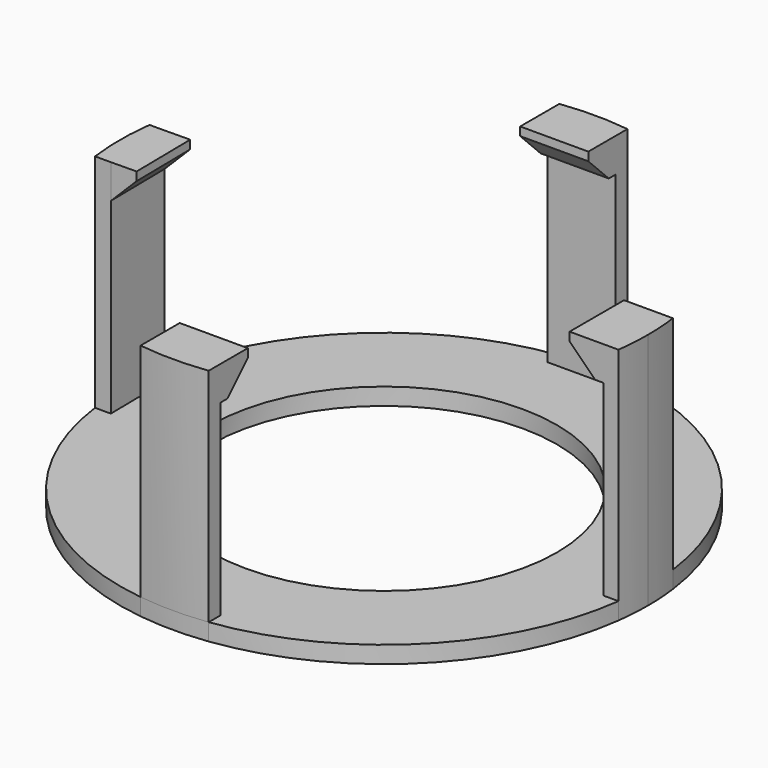
from build123d import *

# Parameters (mm, degrees)
F1_DEPTH  = 14
F0_R      = 10.15
F2_DEPTH  = 1
F3_W      = 4
F3_H      = 2
F4_DEPTH  = 2
F5_SIZE   = 1.5
F6_W      = 4
F6_H      = 2
F7_DEPTH  = 2
F8_SIZE   = 1.5
F9_W      = 4.0003886693
F9_H      = 2
F10_DEPTH = 1.5
F11_SIZE  = 1.49999
F12_W     = 4
F12_H     = 2
F13_DEPTH = 2
F14_SIZE  = 1.5


# Not quite as in the source:
# - a fillet or chamfer is up to 0.001 mm smaller than in the source, because OpenCascade refuses the exact size
# - a feature names something its author has since deleted; it is built from what else it names


with BuildPart() as f1:
    # F0 (on Top) → F1 (new body)
    with BuildSketch(Plane.XY):
        with BuildLine():
            Line((-14.4982938511, 2), (-15.3704261489, 2))
            ThreePointArc((-15.3704261489, 2), (-15.5, 0), (-15.3704261489, -2))
            Line((-15.3704261489, -2), (-14.4425309095, -2))
            Line((-14.4425309095, -2), (-14.4982938511, 2))
        make_face()
    extrude(amount=F1_DEPTH)

    # F9 (on face) → F10 (join)
    with BuildSketch(Plane(origin=(-14.4676006874, -0.2016889929, 0), x_dir=(-0.0139393809, 0.9999028421, 0), z_dir=(0.9999028421, 0.0139393809, 0))):
        with Locations((0.2017085905, 13)):
            Rectangle(F9_W, F9_H)
    extrude(amount=F10_DEPTH)

    # F11 (size 1.5 in the source; OpenCascade refuses exactly that, so slightly less here)
    f11_edges = [f1.edges().sort_by_distance(p)[0] for p in [
        (-12.970558, 0.020909, 12),
    ]]
    chamfer(f11_edges, length=F11_SIZE)


with BuildPart() as f1b:
    # F0 (on Top) → F1, piece 2 (new body)
    with BuildSketch(Plane.XY):
        with BuildLine():
            ThreePointArc((-2, -15.3704261489), (0, -15.5), (2, -15.3704261489))
            Line((2, -15.3704261489), (2, -14.4982938511))
            Line((2, -14.4982938511), (-2, -14.4982938511))
            Line((-2, -14.4982938511), (-2, -15.3704261489))
        make_face()
    extrude(amount=F1_DEPTH)

    # F3 (on face) → F4 (join)
    with BuildSketch(Plane(origin=(0, -14.4982938511, 0), x_dir=(-1, 0, 0), z_dir=(0, 1, 0))):
        with Locations((0, 13)):
            Rectangle(F3_W, F3_H)
    extrude(amount=F4_DEPTH)

    # F5
    f5_edges = [f1b.edges().sort_by_distance(p)[0] for p in [
        (0, -12.498294, 12),
    ]]
    chamfer(f5_edges, length=F5_SIZE)


with BuildPart() as f1c:
    # F0 (on Top) → F1, piece 3 (new body)
    with BuildSketch(Plane.XY):
        with BuildLine():
            Line((2, 14.4982938511), (2, 15.3704261489))
            ThreePointArc((2, 15.3704261489), (0, 15.5), (-2, 15.3704261489))
            Line((-2, 15.3704261489), (-2, 14.4982938511))
            Line((-2, 14.4982938511), (2, 14.4982938511))
        make_face()
    extrude(amount=F1_DEPTH)

    # F6 (on face) → F7 (join)
    with BuildSketch(Plane.XZ.offset(-14.4982938511)):
        with Locations((0, 13)):
            Rectangle(F6_W, F6_H)
    extrude(amount=F7_DEPTH)

    # F8
    f8_edges = [f1c.edges().sort_by_distance(p)[0] for p in [
        (0, 12.498294, 12),
    ]]
    chamfer(f8_edges, length=F8_SIZE)


with BuildPart() as f1d:
    # F0 (on Top) → F1, piece 4 (new body)
    with BuildSketch(Plane.XY):
        with BuildLine():
            ThreePointArc((15.3704261489, -2), (15.4675726167, -1.0020964753), (15.5, 0))
            ThreePointArc((15.5, 0), (15.4675726167, 1.0020964753), (15.3704261489, 2))
            Line((15.3704261489, 2), (14.4982938511, 2))
            Line((14.4982938511, 2), (14.4982938511, -2))
            Line((14.4982938511, -2), (15.3704261489, -2))
        make_face()
    extrude(amount=F1_DEPTH)

    # F12 (on face) → F13 (join)
    with BuildSketch(Plane(origin=(14.4982938511, 0, 0), x_dir=(0, -1, 0), z_dir=(-1, 0, 0))):
        with Locations((0, 13)):
            Rectangle(F12_W, F12_H)
    extrude(amount=F13_DEPTH)

    # F14
    f14_edges = [f1d.edges().sort_by_distance(p)[0] for p in [
        (12.498294, 0, 12),
    ]]
    chamfer(f14_edges, length=F14_SIZE)


with BuildPart() as f2:
    # F0 (on Top) → F2 (new body)
    with BuildSketch(Plane.XY):
        with BuildLine():
            Line((2, 14.4982938511), (2, 15.3704261489))
            ThreePointArc((2, 15.3704261489), (0, 15.5), (-2, 15.3704261489))
            Line((-2, 15.3704261489), (-2, 14.4982938511))
            Line((-2, 14.4982938511), (2, 14.4982938511))
        make_face()
        with BuildLine():
            Line((-14.4982938511, 2), (-15.3704261489, 2))
            ThreePointArc((-15.3704261489, 2), (-15.5, 0), (-15.3704261489, -2))
            Line((-15.3704261489, -2), (-14.4425309095, -2))
            Line((-14.4425309095, -2), (-14.4982938511, 2))
        make_face()
        with BuildLine():
            Line((14.4982938511, 2), (15.3704261489, 2))
            ThreePointArc((15.3704261489, 2), (10.9601551084, 10.9601551084), (2, 15.3704261489))
            Line((2, 15.3704261489), (2, 14.4982938511))
            Line((2, 14.4982938511), (-2, 14.4982938511))
            Line((-2, 14.4982938511), (-2, 15.3704261489))
            ThreePointArc((-2, 15.3704261489), (-10.9601551084, 10.9601551084), (-15.3704261489, 2))
            Line((-15.3704261489, 2), (-14.4982938511, 2))
            Line((-14.4982938511, 2), (-14.4425309095, -2))
            Line((-14.4425309095, -2), (-15.3704261489, -2))
            ThreePointArc((-15.3704261489, -2), (-10.9601551084, -10.9601551084), (-2, -15.3704261489))
            Line((-2, -15.3704261489), (-2, -14.4982938511))
            Line((-2, -14.4982938511), (2, -14.4982938511))
            Line((2, -14.4982938511), (2, -15.3704261489))
            ThreePointArc((2, -15.3704261489), (10.9601551084, -10.9601551084), (15.3704261489, -2))
            Line((15.3704261489, -2), (14.4982938511, -2))
            Line((14.4982938511, -2), (14.4982938511, 2))
        make_face()
        Circle(F0_R, mode=Mode.SUBTRACT)
        with BuildLine():
            ThreePointArc((-2, -15.3704261489), (0, -15.5), (2, -15.3704261489))
            Line((2, -15.3704261489), (2, -14.4982938511))
            Line((2, -14.4982938511), (-2, -14.4982938511))
            Line((-2, -14.4982938511), (-2, -15.3704261489))
        make_face()
    extrude(amount=F2_DEPTH)


solid = Compound([f1.part, f1b.part, f1c.part, f1d.part, f2.part])
